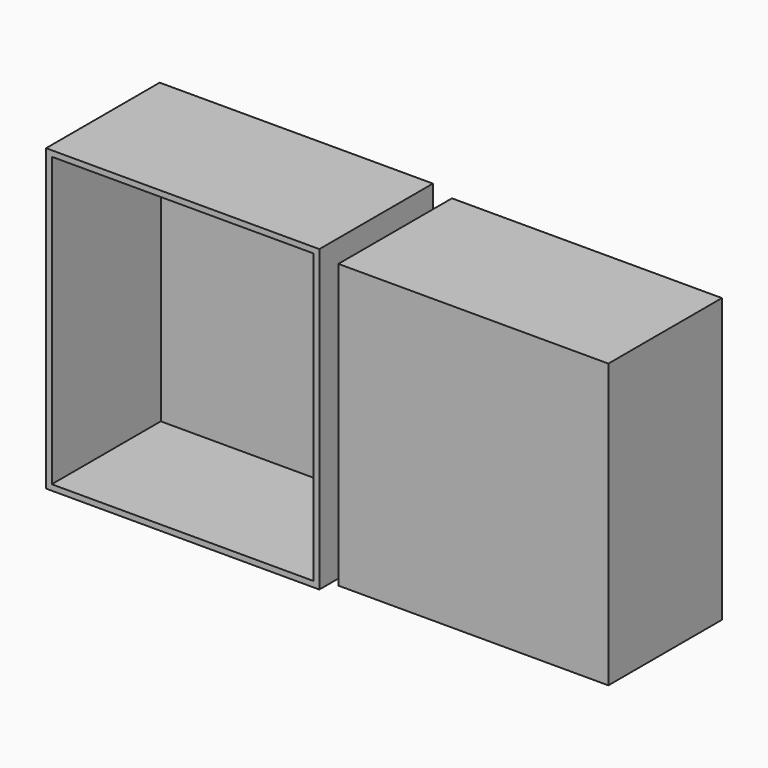
from build123d import *

# Parameters (mm, degrees)
F0_W     = 122.2361847758
F0_H     = 134.0652927756
F5_DEPTH = 63.5
F6_T     = -2.54
F1_W     = 120.766825974
F1_H     = 126.7148703337
F2_DEPTH = 63.5


# Not quite as in the source:
# - the program builds the solid bodies; features that only make, move or delete a surface that nothing else refers to are left out


with BuildPart() as f5:
    # F0 (on Front) → F5 (new body)
    with BuildSketch(Plane.XZ):
        with Locations((0.2992935479, 0.6186775863)):
            Rectangle(F0_W, F0_H)
    extrude(amount=F5_DEPTH)

    # F6
    f6_openings = [f5.faces().sort_by_distance(p)[0] for p in [
        (0.299294, -63.5, 0.618678),
    ]]
    offset(amount=F6_T, openings=f6_openings)


with BuildPart() as f2:
    # F1 (on Front) → F2 (new body)
    with BuildSketch(Plane.XZ):
        with Locations((130.3160600364, 1.2532249093)):
            Rectangle(F1_W, F1_H)
    extrude(amount=F2_DEPTH)


solid = Compound([f5.part, f2.part])
